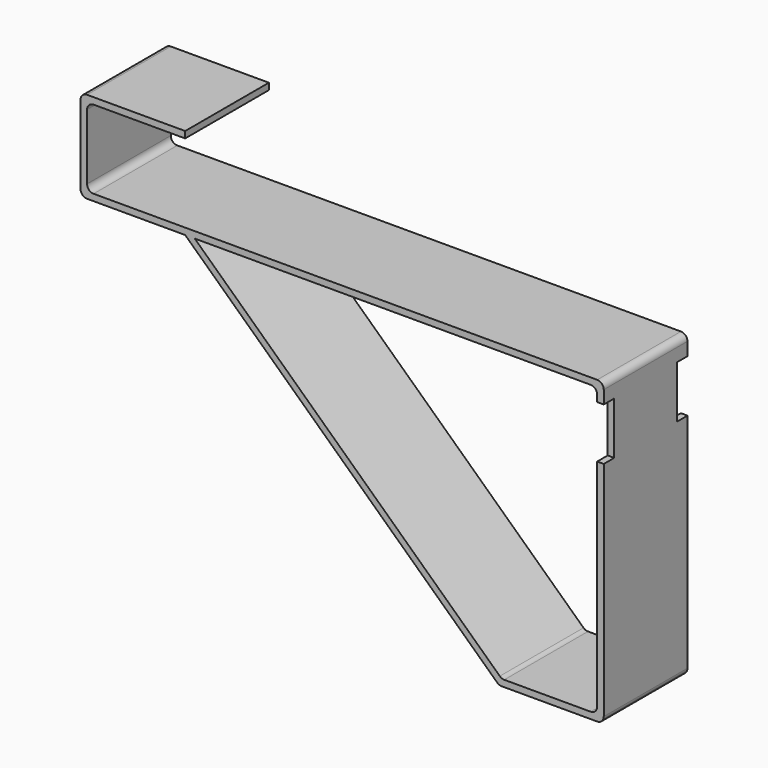
from build123d import *

# Parameters (mm, degrees)
F1_DEPTH = 50.8
F2_R     = 3.175
F4_W     = 6.35
F4_H     = 25.4
F5_DEPTH = 25.4


# Not quite as in the source:
# - two fillets or chamfers of one size are made in one step
# - a feature names something its author has since deleted; it is built from what else it names


with BuildPart() as f1:
    # F0 (on Front) → F1 (new body)
    with BuildSketch(Plane.XZ):
        Polygon((89.9496172311, 43.3501401251), (-160.8753827689, 43.3501401251), (-160.8753827689, 81.4501401251), (-113.2503827689, 81.4501401251), (-113.2503827689, 84.6251401251), (-164.0503827689, 84.6251401251), (-164.0503827689, 40.1751401251), (-113.2503827689, 40.1751401251), (39.1496172311, -102.6998598749), (89.9496172311, -102.6998598749), align=None)
        Polygon((-108.6081703534, 40.1751401251), (86.7746172311, 40.1751401251), (86.7746172311, -99.5248598749), (40.4051629799, -99.5248598749), align=None, mode=Mode.SUBTRACT)
    extrude(amount=F1_DEPTH)

    # F2
    f2_edges = [f1.edges().sort_by_distance(p)[0] for p in [
        (-164.050383, -25.4, 84.62514),
        (-160.875383, -25.4, 43.35014),
        (89.949617, -25.4, 43.35014),
        (89.949617, -25.4, -102.69986),
        (-164.050383, -25.4, 40.17514),
        (-160.875383, -25.4, 81.45014),
        (39.149617, -25.4, -102.69986),
        (40.405163, -25.4, -99.52486),
        (86.774617, -25.4, 40.17514),
        (86.774617, -25.4, -99.52486),
    ]]
    fillet(f2_edges, radius=F2_R)

    # F4 (on face) → F5 (cut)
    with BuildSketch(Plane.YZ.offset(89.9496172311)):
        with Locations((-3.175, 21.1251401251)):
            Rectangle(F4_W, F4_H)
        with Locations((-47.625, 21.1251401251)):
            Rectangle(F4_W, F4_H)
    extrude(amount=-F5_DEPTH, mode=Mode.SUBTRACT)


solid = f1.part
